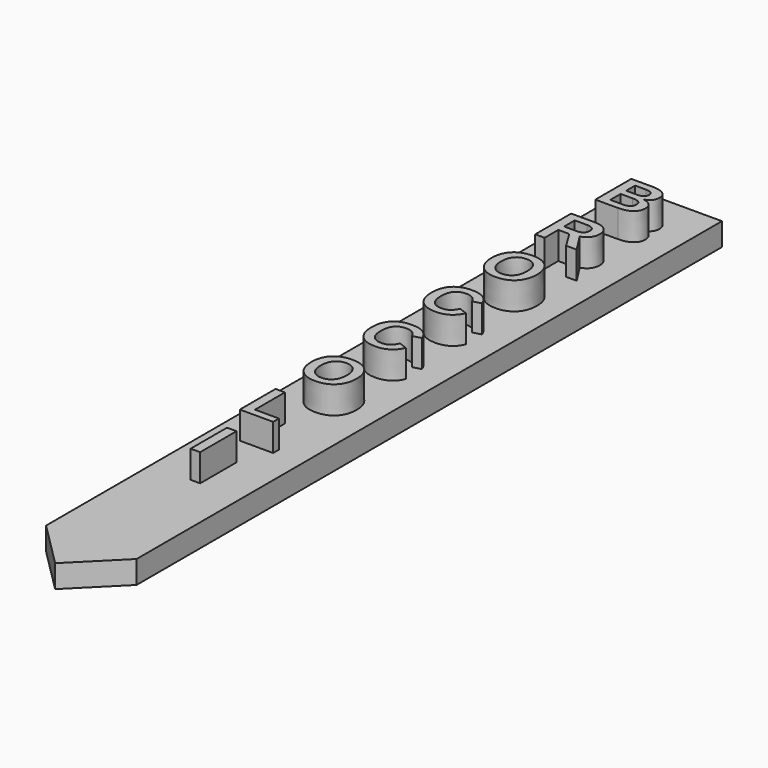
from build123d import *

# Parameters (mm, degrees)
F1_DEPTH       = 2.5
F2_TEXT_SIZE   = 7.1414709878
F2_TEXT_SIZE_2 = 7.2272830746
F2_TEXT_SIZE_3 = 7.0972342251
F3_DEPTH       = 3


# Not quite as in the source:
# - Text() gives the source's letters only with a copy of the font that has no kerning and outlines rounded to 1/6400 em; it was checked with that copy


with BuildPart() as f1:
    # F0 (on Top) → F1 (new body)
    with BuildSketch(Plane.XY):
        Polygon((-4.9497474683, 4.9497474683), (0, 0), (4.9497474683, 4.9497474683), (4.9497474683, 84.9497474683), (-4.9497474683, 84.9497474683), align=None)
    extrude(amount=F1_DEPTH)

    # F2 (on face) → F3 (join)
    with BuildSketch(Plane.XY.offset(2.5)):
        with Locations((-2.8579389353, 76.8078883571)):
            Text('B', F2_TEXT_SIZE, font='Arimo', font_style=FontStyle.BOLD, text_align=(TextAlign.LEFT, TextAlign.BOTTOM))
        with Locations((-2.8579389353, 68.5951967212)):
            Text('R', F2_TEXT_SIZE, font='Arimo', font_style=FontStyle.BOLD, text_align=(TextAlign.LEFT, TextAlign.BOTTOM))
        with Locations((-2.8579389353, 60.3825050852)):
            Text('O', F2_TEXT_SIZE, font='Arimo', font_style=FontStyle.BOLD, text_align=(TextAlign.LEFT, TextAlign.BOTTOM))
        with Locations((-2.8579389353, 52.1698134493)):
            Text('C', F2_TEXT_SIZE, font='Arimo', font_style=FontStyle.BOLD, text_align=(TextAlign.LEFT, TextAlign.BOTTOM))
        with Locations((-2.8579389353, 43.9571218133)):
            Text('C', F2_TEXT_SIZE, font='Arimo', font_style=FontStyle.BOLD, text_align=(TextAlign.LEFT, TextAlign.BOTTOM))
        with Locations((-2.8579389353, 35.7444301774)):
            Text('O', F2_TEXT_SIZE, font='Arimo', font_style=FontStyle.BOLD, text_align=(TextAlign.LEFT, TextAlign.BOTTOM))
        with Locations((-1.0761503185, 19.2601736635)):
            Text('I', F2_TEXT_SIZE_2, font='Arimo', font_style=FontStyle.BOLD, text_align=(TextAlign.LEFT, TextAlign.BOTTOM))
        with Locations((-2.3049377089, 27.5331865996)):
            Text('L', F2_TEXT_SIZE_3, font='Arimo', font_style=FontStyle.BOLD, text_align=(TextAlign.LEFT, TextAlign.BOTTOM))
    extrude(amount=F3_DEPTH)


solid = f1.part
